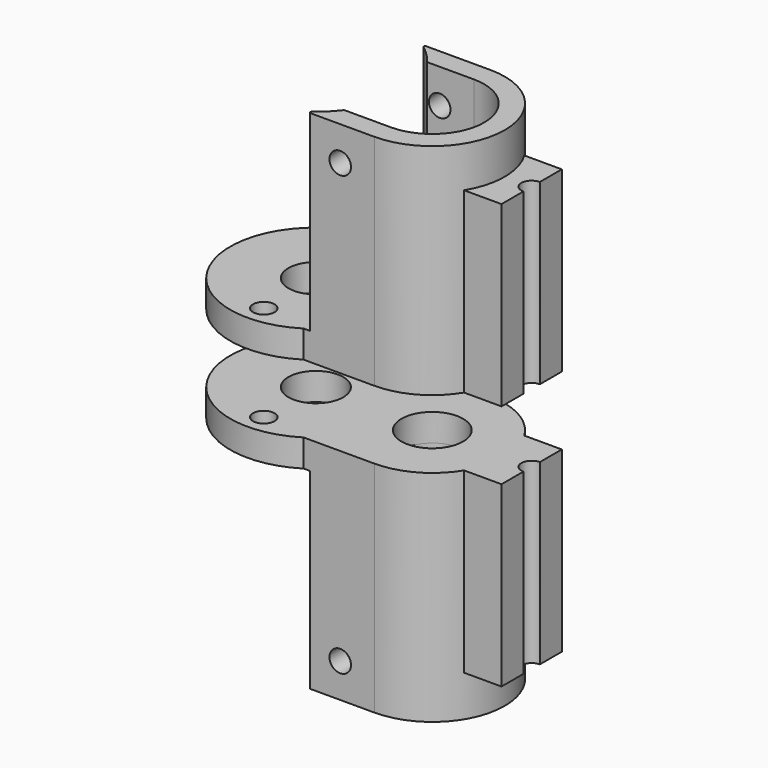
from build123d import *

# Parameters (mm, degrees)
F2_R         = 1.575
F2_R_2       = 4
F2_R_3       = 4.5
F4_DEPTH     = 4
F6_DEPTH     = 4
F8_DEPTH     = 24
F9_R         = 1.575
F10_DEPTH    = 23.076
F11_DEPTH    = 22
F12_T1_DEPTH = 29.5834567143
F12_T3_DEPTH = 6.0635066478


# Not quite as in the source:
# - a fillet or chamfer that OpenCascade refuses, or shapes differently, is made with other operations: its cross-section is extruded or revolved along the edge and cut away or added


with BuildPart() as f4:
    # F2 (on Top) → F4 (new body)
    with BuildSketch(Plane.XY):
        with BuildLine():
            ThreePointArc((26.0321993446, 5.5), (22.1801604705, 9.2193580308), (17, 10.575))
            Line((17, 10.575), (6.6647861931, 10.575))
            ThreePointArc((6.6647861931, 10.575), (-12.5, 0), (6.6647861931, -10.575))
            Line((6.6647861931, -10.575), (17, -10.575))
            ThreePointArc((17, -10.575), (22.1801604705, -9.2193580308), (26.0321993446, -5.5))
            Line((26.0321993446, -5.5), (31.5, -5.5))
            Line((31.5, -5.5), (31.5, -1.5))
            ThreePointArc((31.5, -1.5), (30, 0), (31.5, 1.5))
            Line((31.5, 1.5), (31.5, 5.5))
            Line((31.5, 5.5), (26.0321993446, 5.5))
        make_face()
        with Locations((0, -9.5)):
            Circle(F2_R, mode=Mode.SUBTRACT)
        Circle(F2_R_2, mode=Mode.SUBTRACT)
        with Locations((0, 9.5)):
            Circle(F2_R, mode=Mode.SUBTRACT)
        with Locations((17, 0)):
            Circle(F2_R_3, mode=Mode.SUBTRACT)
    extrude(amount=F4_DEPTH)

    # F5 (on face) → F6 (join)
    with BuildSketch(Plane.XY.offset(4)):
        with BuildLine():
            ThreePointArc((12.6482352941, 1.1454885179), (17.5775200531, 4.4627873116), (21.5, 0))
            ThreePointArc((21.5, 0), (17.5775200531, -4.4627873116), (12.6482352941, -1.1454885179))
            ThreePointArc((12.6482352941, -1.1454885179), (10.9116487762, -6.498147504), (7.0327359541, -10.575))
            Line((7.0327359541, -10.575), (17, -10.575))
            ThreePointArc((17, -10.575), (22.1801604705, -9.2193580308), (26.0321993446, -5.5))
            ThreePointArc((26.0321993446, -5.5), (27.575, 0), (26.0321993446, 5.5))
            ThreePointArc((26.0321993446, 5.5), (22.1801604705, 9.2193580308), (17, 10.575))
            Line((17, 10.575), (7.0327359541, 10.575))
            ThreePointArc((7.0327359541, 10.575), (10.9116487762, 6.498147504), (12.6482352941, 1.1454885179))
        make_face()
    extrude(amount=F6_DEPTH)

    # F7 (on face) → F8 (join)
    with BuildSketch(Plane.XY.offset(8)):
        with BuildLine():
            Line((10.1935948026, 7.575), (17, 7.575))
            ThreePointArc((17, 7.575), (24.575, 0), (17, -7.575))
            Line((17, -7.575), (10.1935948026, -7.575))
            ThreePointArc((10.1935948026, -7.575), (8.7428037742, -9.2115895569), (7.0327359541, -10.575))
            Line((7.0327359541, -10.575), (17, -10.575))
            ThreePointArc((17, -10.575), (27.575, 0), (17, 10.575))
            Line((17, 10.575), (7.0327359541, 10.575))
            ThreePointArc((7.0327359541, 10.575), (8.7428037742, 9.2115895569), (10.1935948026, 7.575))
        make_face()
    extrude(amount=F8_DEPTH)

    # F9 (on face) → F10 (cut, through all)
    with BuildSketch(Plane.XZ.offset(10.575)):
        with Locations((12.016367977, 27)):
            Circle(F9_R)
    extrude(amount=-F10_DEPTH, mode=Mode.SUBTRACT)

    # F5 (on face) → F11 (join)
    with BuildSketch(Plane.XY.offset(4)):
        with BuildLine():
            Line((31.5, 5.5), (26.0321993446, 5.5))
            ThreePointArc((26.0321993446, 5.5), (27.575, 0), (26.0321993446, -5.5))
            Line((26.0321993446, -5.5), (31.5, -5.5))
            Line((31.5, -5.5), (31.5, -1.5))
            ThreePointArc((31.5, -1.5), (30, 0), (31.5, 1.5))
            Line((31.5, 1.5), (31.5, 5.5))
        make_face()
    extrude(amount=F11_DEPTH)

    # F12: fillet of radius 0.2 on 4 edges, made by hand

    # F12_s2 → F12_t1 (cut)
    with BuildSketch(Plane.XY.offset(4)):
        with BuildLine():
            ThreePointArc((7.5472640873, -10.2141472868), (7.4761574035, -10.4375677927), (7.6661186398, -10.575))
            Line((7.6661186398, -10.575), (7.0327359541, -10.575))
            ThreePointArc((7.0327359541, -10.575), (7.2922324409, -10.3977567787), (7.5472640873, -10.2141472868))
        make_face()
        with BuildLine():
            ThreePointArc((7.6661186398, 10.575), (7.4761574035, 10.4375677927), (7.5472640873, 10.2141472868))
            ThreePointArc((7.5472640873, 10.2141472868), (7.2922324409, 10.3977567787), (7.0327359541, 10.575))
            Line((7.0327359541, 10.575), (7.6661186398, 10.575))
        make_face()
    extrude(amount=F12_T1_DEPTH, mode=Mode.SUBTRACT)

    # F12_s4 → F12_t3 (cut)
    with BuildSketch(Plane.XY.offset(4)):
        with BuildLine():
            ThreePointArc((12.9257822278, 1.9106934722), (12.7164808258, 1.7976148331), (12.5471135431, 1.9646734428))
            ThreePointArc((12.5471135431, 1.9646734428), (12.6043312691, 1.5559027147), (12.6482352941, 1.1454885179))
            ThreePointArc((12.6482352941, 1.1454885179), (12.769671427, 1.5343794069), (12.9257822278, 1.9106934722))
        make_face()
        with BuildLine():
            ThreePointArc((12.5471135431, -1.9646734428), (12.7164808258, -1.7976148331), (12.9257822278, -1.9106934722))
            ThreePointArc((12.9257822278, -1.9106934722), (12.769671427, -1.5343794069), (12.6482352941, -1.1454885179))
            ThreePointArc((12.6482352941, -1.1454885179), (12.6043312691, -1.5559027147), (12.5471135431, -1.9646734428))
        make_face()
    extrude(amount=F12_T3_DEPTH, mode=Mode.SUBTRACT)


with BuildPart() as f4_1:
    # F13: moved
    add(f4.part.moved(Location((0, 0, 5))))


with BuildPart() as f14_1:
    # F14: instance of F4
    add(f4_1.part.mirror(Plane.XY))


solid = Compound([f4_1.part, f14_1.part])
